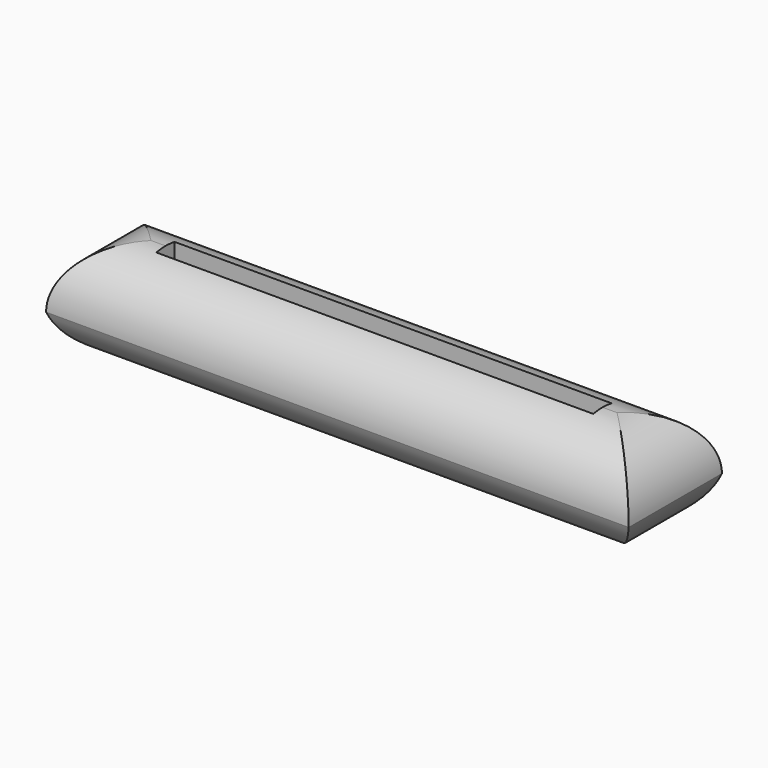
from build123d import *

# Parameters (mm, degrees)
F0_W        = 50.8
F0_H        = 10.16
F0_W_2      = 38.1
F0_H_2      = 2
F1_DEPTH    = 8.636
F2_T1_DEPTH = 35.56
F2_T3_DEPTH = 76.2
F3_T1_DEPTH = 34.390055716
F3_T3_DEPTH = 75.030055716


# Not quite as in the source:
# - a fillet or chamfer that OpenCascade refuses, or shapes differently, is made with other operations: its cross-section is extruded or revolved along the edge and cut away or added


with BuildPart() as f1:
    # F0 (on Top) → F1 (new body)
    with BuildSketch(Plane.XY):
        Rectangle(F0_W, F0_H)
        Rectangle(F0_W_2, F0_H_2, mode=Mode.SUBTRACT)
    extrude(amount=F1_DEPTH)

    # F2: fillet of radius 5.08 on 4 edges, made by hand

    # F2_s2 → F2_t1 (cut)
    with BuildSketch(Plane.XZ.offset(-17.78)):
        with BuildLine():
            ThreePointArc((-25.4, 3.556), (-23.9121024484, 7.1481024484), (-20.32, 8.636))
            Line((-20.32, 8.636), (-25.4, 8.636))
            Line((-25.4, 8.636), (-25.4, 3.556))
        make_face()
        with BuildLine():
            ThreePointArc((25.4, 3.556), (23.9121024484, 7.1481024484), (20.32, 8.636))
            Line((20.32, 8.636), (25.4, 8.636))
            Line((25.4, 8.636), (25.4, 3.556))
        make_face()
    extrude(amount=F2_T1_DEPTH, mode=Mode.SUBTRACT)

    # F2_s4 → F2_t3 (cut)
    with BuildSketch(Plane.YZ.offset(-38.1)):
        with BuildLine():
            ThreePointArc((-5.08, 3.556), (-3.5921024484, 7.1481024484), (0, 8.636))
            Line((0, 8.636), (-5.08, 8.636))
            Line((-5.08, 8.636), (-5.08, 3.556))
        make_face()
        with BuildLine():
            ThreePointArc((5.08, 3.556), (3.5921024484, 7.1481024484), (0, 8.636))
            Line((0, 8.636), (5.08, 8.636))
            Line((5.08, 8.636), (5.08, 3.556))
        make_face()
    extrude(amount=F2_T3_DEPTH, mode=Mode.SUBTRACT)

    # F3: fillet of radius 5.08 on 4 edges, made by hand

    # F3_s2 → F3_t1 (cut)
    with BuildSketch(Plane.XZ.offset(-17.195027858)):
        with BuildLine():
            ThreePointArc((-20.5539888568, 0), (-23.5593573866, 0.9843730639), (-25.4, 3.556))
            Line((-25.4, 3.556), (-25.4, 0))
            Line((-25.4, 0), (-20.5539888568, 0))
        make_face()
        with BuildLine():
            ThreePointArc((20.5539888568, 0), (23.5593573866, 0.9843730639), (25.4, 3.556))
            Line((25.4, 3.556), (25.4, 0))
            Line((25.4, 0), (20.5539888568, 0))
        make_face()
    extrude(amount=F3_T1_DEPTH, mode=Mode.SUBTRACT)

    # F3_s4 → F3_t3 (cut)
    with BuildSketch(Plane.YZ.offset(-37.515027858)):
        with BuildLine():
            ThreePointArc((-5.08, 3.556), (-3.2393573866, 0.9843730639), (-0.2339888568, 0))
            Line((-0.2339888568, 0), (-5.08, 0))
            Line((-5.08, 0), (-5.08, 3.556))
        make_face()
        with BuildLine():
            ThreePointArc((0.2339888568, 0), (3.2393573866, 0.9843730639), (5.08, 3.556))
            Line((5.08, 3.556), (5.08, 0))
            Line((5.08, 0), (0.2339888568, 0))
        make_face()
    extrude(amount=F3_T3_DEPTH, mode=Mode.SUBTRACT)


solid = f1.part
